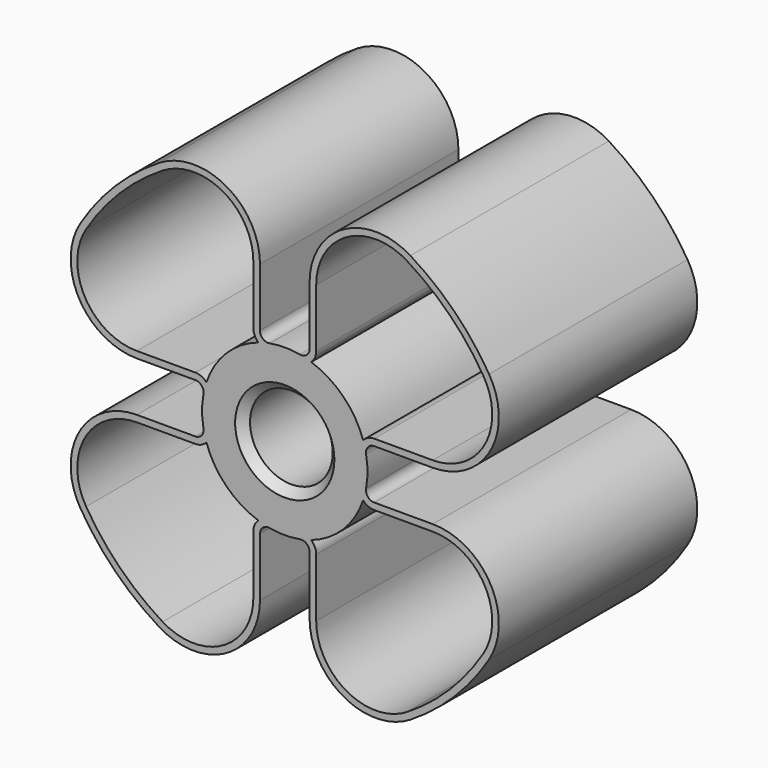
from build123d import *

# Parameters (mm, degrees)
F0_R      = 10
F0_R_2    = 5
F1_DEPTH  = 30
F2_R      = 29
F2_R_2    = 10
F3_DEPTH  = 30
F5_DEPTH  = 30.001
F6_R      = 8
F7_R      = 1
F8_T      = -0.8
F9_DEPTH  = 25
F10_R     = 5.8
F10_R_2   = 5
F11_DEPTH = 30
F12_SIZE  = 1


with BuildPart() as f1:
    # F0 (on Front) → F1 (new body)
    with BuildSketch(Plane.XZ):
        Circle(F0_R)
        Circle(F0_R_2, mode=Mode.SUBTRACT)
    extrude(amount=F1_DEPTH)

    # F2 (on face) → F3 (join, through all)
    with BuildSketch(Plane.XZ.offset(30)):
        Circle(F2_R)
        Circle(F2_R_2, mode=Mode.SUBTRACT)
    extrude(amount=-F3_DEPTH)

    # F4 (on face) → F5 (cut, through all)
    with BuildSketch(Plane.XZ.offset(30)):
        with BuildLine():
            ThreePointArc((-9.5393920142, -3), (-10, 0), (-9.5393920142, 3))
            Line((-9.5393920142, 3), (-32.1717076004, 3))
            Line((-32.1717076004, 3), (-32.1717076004, -3))
            Line((-32.1717076004, -3), (-9.5393920142, -3))
        make_face()
        with BuildLine():
            Line((-3, -33.598061651), (3, -33.598061651))
            Line((3, -33.598061651), (3, -9.5393920142))
            ThreePointArc((3, -9.5393920142), (0, -10), (-3, -9.5393920142))
            Line((-3, -9.5393920142), (-3, -33.598061651))
        make_face()
        with BuildLine():
            Line((3, 9.5393920142), (3, 33.598061651))
            Line((3, 33.598061651), (-3, 33.598061651))
            Line((-3, 33.598061651), (-3, 9.5393920142))
            ThreePointArc((-3, 9.5393920142), (0, 10), (3, 9.5393920142))
        make_face()
        with BuildLine():
            Line((9.5393920142, -3), (32.1717076004, -3))
            Line((32.1717076004, -3), (32.1717076004, 3))
            Line((32.1717076004, 3), (9.5393920142, 3))
            ThreePointArc((9.5393920142, 3), (10, 0), (9.5393920142, -3))
        make_face()
    extrude(amount=-F5_DEPTH, mode=Mode.SUBTRACT)

    # F6
    f6_edges = [f1.edges().sort_by_distance(p)[0] for p in [
        (-3, -15, 28.84441),
        (-28.84441, -15, 3),
        (-28.84441, -15, -3),
        (3, -15, 28.84441),
        (-3, -15, -28.84441),
        (3, -15, -28.84441),
        (28.84441, -15, -3),
        (28.84441, -15, 3),
    ]]
    fillet(f6_edges, radius=F6_R)

    # F7
    f7_edges = [f1.edges().sort_by_distance(p)[0] for p in [
        (-9.539392, -15, 3),
        (-9.539392, -15, -3),
        (-3, -15, -9.539392),
        (3, -15, -9.539392),
        (9.539392, -15, 3),
        (9.539392, -15, -3),
        (-3, -15, 9.539392),
        (3, -15, 9.539392),
    ]]
    fillet(f7_edges, radius=F7_R)

    # F8
    f8_openings = [f1.faces().sort_by_distance(p)[0] for p in [
        (14.352599, -30, 3.732239),
    ]]
    offset(amount=F8_T, openings=f8_openings)

    # F9 (cut): faces of the model
    f9_faces = [f1.faces().sort_by_distance(p)[0] for p in [
        (14.3525988232, -0.8, 4.5096111786),
        (14.3525988232, -0.8, 4.5096111786),
        (14.3525988232, -0.8, 4.5096111786),
        (14.3525988232, -0.8, 4.5096111786),
    ]]
    extrude(f9_faces, amount=-F9_DEPTH, mode=Mode.SUBTRACT)

    # F10 (on face) → F11 (join, through all)
    with BuildSketch(Plane.XZ.offset(30)):
        with BuildLine():
            ThreePointArc((9.0466559275, 1.6727272727), (9.083408006, 2.4856530923), (9.4744050932, 3.1993199482))
            ThreePointArc((9.4744050932, 3.1993199482), (7.0710678119, 7.0710678119), (3.1993199482, 9.4744050932))
            ThreePointArc((3.1993199482, 9.4744050932), (2.4856530923, 9.083408006), (1.6727272727, 9.0466559275))
            ThreePointArc((1.6727272727, 9.0466559275), (0, 9.2), (-1.6727272727, 9.0466559275))
            ThreePointArc((-1.6727272727, 9.0466559275), (-2.4856530923, 9.083408006), (-3.1993199482, 9.4744050932))
            ThreePointArc((-3.1993199482, 9.4744050932), (-7.0710678119, 7.0710678119), (-9.4744050932, 3.1993199482))
            ThreePointArc((-9.4744050932, 3.1993199482), (-9.083408006, 2.4856530923), (-9.0466559275, 1.6727272727))
            ThreePointArc((-9.0466559275, 1.6727272727), (-9.2, 0), (-9.0466559275, -1.6727272727))
            ThreePointArc((-9.0466559275, -1.6727272727), (-9.083408006, -2.4856530923), (-9.4744050932, -3.1993199482))
            ThreePointArc((-9.4744050932, -3.1993199482), (-7.0710678119, -7.0710678119), (-3.1993199482, -9.4744050932))
            ThreePointArc((-3.1993199482, -9.4744050932), (-2.4856530923, -9.083408006), (-1.6727272727, -9.0466559275))
            ThreePointArc((-1.6727272727, -9.0466559275), (0, -9.2), (1.6727272727, -9.0466559275))
            ThreePointArc((1.6727272727, -9.0466559275), (2.4856530923, -9.083408006), (3.1993199482, -9.4744050932))
            ThreePointArc((3.1993199482, -9.4744050932), (7.0710678119, -7.0710678119), (9.4744050932, -3.1993199482))
            ThreePointArc((9.4744050932, -3.1993199482), (9.083408006, -2.4856530923), (9.0466559275, -1.6727272727))
            ThreePointArc((9.0466559275, -1.6727272727), (9.2, 0), (9.0466559275, 1.6727272727))
        make_face()
        Circle(F10_R, mode=Mode.SUBTRACT)
        Circle(F10_R)
        Circle(F10_R_2, mode=Mode.SUBTRACT)
    extrude(amount=-F11_DEPTH)

    # F12
    f12_edges = [f1.edges().sort_by_distance(p)[0] for p in [
        (5, -15, 0),
        (-5, 0, 0),
        (-5, -30, 0),
    ]]
    chamfer(f12_edges, length=F12_SIZE)


solid = f1.part
